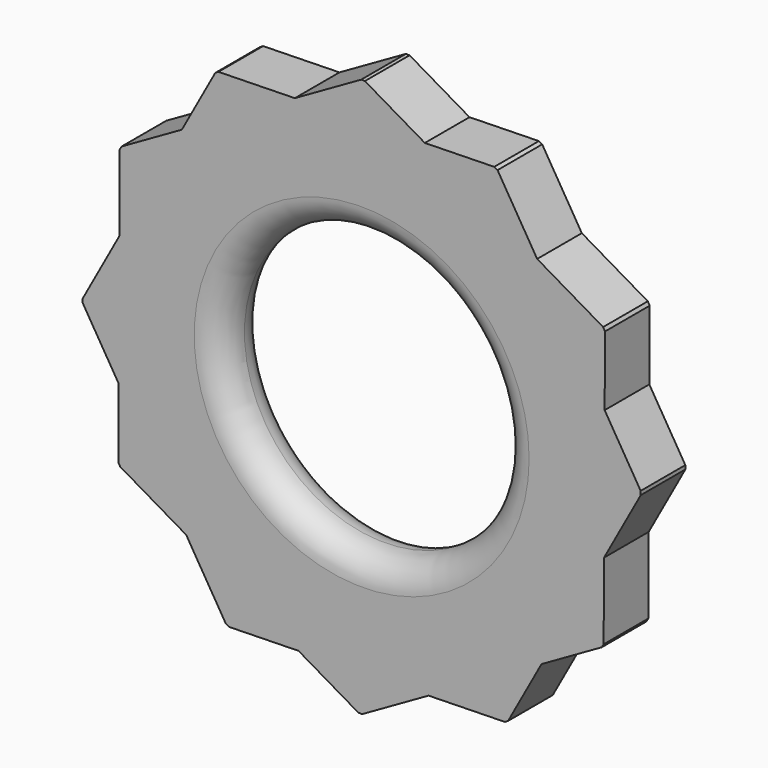
from build123d import *

# Parameters (mm, degrees)
F0_R     = 6.35
F1_DEPTH = 2.54
F2_R     = 1.26999


# Not quite as in the source:
# - a fillet or chamfer is up to 0.001 mm smaller than in the source, because OpenCascade refuses the exact size


with BuildPart() as f1:
    # F0 (on Front) → F1 (new body)
    with BuildSketch(Plane.XZ):
        Polygon((8.1817057439, -8.042901042), (11.0273133855, -2.8538767742), (11.0562094944, 3.0641144995), (7.9851864785, 8.1229951402), (2.8745037505, 11.1070155415), (-3.042126907, 10.9768719144), (-8.1817057439, 8.042901042), (-11.0273133855, 2.8538767742), (-11.0562094944, -3.0641144995), (-7.9851864785, -8.1229951402), (-2.8745037505, -11.1070155415), (3.042126907, -10.9768719144), align=None)
        Circle(F0_R, mode=Mode.SUBTRACT)
        with BuildLine():
            Line((-3.042126907, 10.9768719144), (2.8745037505, 11.1070155415))
            Line((2.8745037505, 11.1070155415), (0.1476963834, 12.6991411433))
            ThreePointArc((0.1476963834, 12.6991411433), (0.0620102654, 12.6998486104), (-0.0236786756, 12.699977926))
            Line((-0.0236786756, 12.699977926), (-3.042126907, 10.9768719144))
        make_face()
        with BuildLine():
            Line((-8.1817057439, 8.042901042), (-3.042126907, 10.9768719144))
            Line((-3.042126907, 10.9768719144), (-6.5169336782, 10.9004392312))
            ThreePointArc((-6.5169336782, 10.9004392312), (-6.5903320193, 10.8562205152), (-6.6634303404, 10.8115075775))
            Line((-6.6634303404, 10.8115075775), (-8.1817057439, 8.042901042))
        make_face()
        with BuildLine():
            Line((-11.0273133855, 2.8538767742), (-8.1817057439, 8.042901042))
            Line((-8.1817057439, 8.042901042), (-10.9239306447, 6.4774793917))
            ThreePointArc((-10.9239306447, 6.4774793917), (-10.9673863881, 6.4036267703), (-11.0103428492, 6.3294826284))
            Line((-11.0103428492, 6.3294826284), (-11.0273133855, 2.8538767742))
        make_face()
        with BuildLine():
            Line((-12.6947553855, -0.3649461623), (-11.0562094944, -3.0641144995))
            Line((-11.0562094944, -3.0641144995), (-11.0273133855, 2.8538767742))
            Line((-11.0273133855, 2.8538767742), (-12.6985241258, -0.1936105045))
            ThreePointArc((-12.6985241258, -0.1936105045), (-12.6969287649, -0.2792846905), (-12.6947553855, -0.3649461623))
        make_face()
        with BuildLine():
            Line((-10.9866641736, -6.3704952976), (-7.9851864785, -8.1229951402))
            Line((-7.9851864785, -8.1229951402), (-11.0562094944, -3.0641144995))
            Line((-11.0562094944, -3.0641144995), (-11.0716270281, -6.2216617516))
            ThreePointArc((-11.0716270281, -6.2216617516), (-11.0293966535, -6.2962218401), (-10.9866641736, -6.3704952976))
        make_face()
        with BuildLine():
            Line((-6.0313250452, -11.1764537399), (-2.8745037505, -11.1070155415))
            Line((-2.8745037505, -11.1070155415), (-7.9851864785, -8.1229951402))
            Line((-7.9851864785, -8.1229951402), (-6.1815904476, -11.0940497357))
            ThreePointArc((-6.1815904476, -11.0940497357), (-6.1065967456, -11.1355052057), (-6.0313250452, -11.1764537399))
        make_face()
        with BuildLine():
            Line((0.0236786756, -12.699977926), (3.042126907, -10.9768719144))
            Line((3.042126907, -10.9768719144), (-2.8745037505, -11.1070155415))
            Line((-2.8745037505, -11.1070155415), (-0.1476963834, -12.6991411433))
            ThreePointArc((-0.1476963834, -12.6991411433), (-0.0620102654, -12.6998486104), (0.0236786756, -12.699977926))
        make_face()
        with BuildLine():
            Line((6.6634303404, -10.8115075775), (8.1817057439, -8.042901042))
            Line((8.1817057439, -8.042901042), (3.042126907, -10.9768719144))
            Line((3.042126907, -10.9768719144), (6.5169336782, -10.9004392312))
            ThreePointArc((6.5169336782, -10.9004392312), (6.5903320193, -10.8562205152), (6.6634303404, -10.8115075775))
        make_face()
        with BuildLine():
            ThreePointArc((10.9239306447, -6.4774793917), (10.9673863881, -6.4036267703), (11.0103428492, -6.3294826284))
            Line((11.0103428492, -6.3294826284), (11.0273133855, -2.8538767742))
            Line((11.0273133855, -2.8538767742), (8.1817057439, -8.042901042))
            Line((8.1817057439, -8.042901042), (10.9239306447, -6.4774793917))
        make_face()
        with BuildLine():
            Line((11.0273133855, -2.8538767742), (12.6985241258, 0.1936105045))
            ThreePointArc((12.6985241258, 0.1936105045), (12.6969287649, 0.2792846905), (12.6947553855, 0.3649461623))
            Line((12.6947553855, 0.3649461623), (11.0562094944, 3.0641144995))
            Line((11.0562094944, 3.0641144995), (11.0273133855, -2.8538767742))
        make_face()
        with BuildLine():
            Line((11.0562094944, 3.0641144995), (11.0716270281, 6.2216617516))
            ThreePointArc((11.0716270281, 6.2216617516), (11.0293966535, 6.2962218401), (10.9866641736, 6.3704952976))
            Line((10.9866641736, 6.3704952976), (7.9851864785, 8.1229951402))
            Line((7.9851864785, 8.1229951402), (11.0562094944, 3.0641144995))
        make_face()
        with BuildLine():
            Line((2.8745037505, 11.1070155415), (7.9851864785, 8.1229951402))
            Line((7.9851864785, 8.1229951402), (6.1815904476, 11.0940497357))
            ThreePointArc((6.1815904476, 11.0940497357), (6.1065967456, 11.1355052057), (6.0313250452, 11.1764537399))
            Line((6.0313250452, 11.1764537399), (2.8745037505, 11.1070155415))
        make_face()
    extrude(amount=F1_DEPTH)

    # F2 (radius 1.27 in the source; OpenCascade refuses exactly that, so slightly less here)
    f2_edges = [f1.edges().sort_by_distance(p)[0] for p in [
        (-6.35, -2.54, 0),
        (-6.35, 0, 0),
    ]]
    fillet(f2_edges, radius=F2_R)


solid = f1.part
